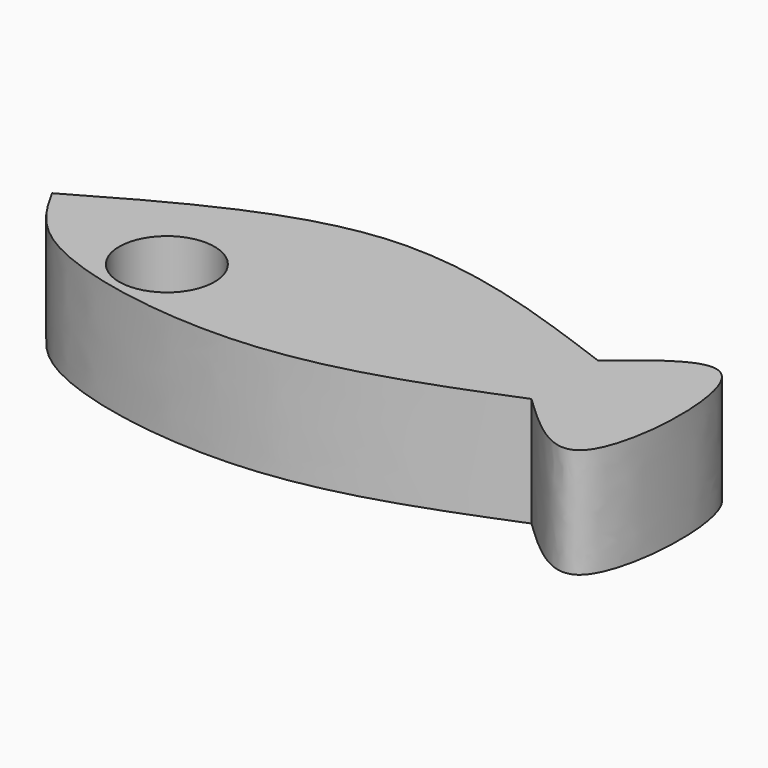
from build123d import *

# Parameters (mm, degrees)
F1_DEPTH = 11.684
F3_D     = 10.16


with BuildPart() as f1:
    # F0 (on Top) → F1 (new body)
    with BuildSketch(Plane.XY):
        with BuildLine():
            add(Edge.make_bspline(
                [(-36.1180268228, 4.0337503888), (-27.3021805537, 9.101057148), (-9.7698211862, 19.1785744295), (8.9001535273, 12.2858719608), (18.1822516024, 8.8590467349)],
                knots=[0, 0, 0, 0, 0.5028328523, 1, 1, 1, 1], degree=3))
            add(Edge.make_bspline(
                [(-36.1180268228, 4.0337503888), (-34.7839596362, 1.6128883032), (-31.2635443087, -4.7754256271), (-5.5172595701, -9.5463141676), (10.1612689912, -3.2309029238), (18.1822516024, 0)],
                knots=[0, 0, 0, 0, 0.2295947399, 0.6058681674, 1, 1, 1, 1], degree=3))
            add(Edge.make_bspline(
                [(18.1822516024, 8.8590467349), (22.0562457427, 12.1275590602), (30.9221363084, 19.6077646412), (29.7113094866, -10.9758153664), (21.6541939321, -3.3053349507), (18.1822516024, 0)],
                knots=[0, 0, 0, 0, 0.3063461125, 0.7010932414, 1, 1, 1, 1], degree=3))
        make_face()
    extrude(amount=F1_DEPTH)

    # F3 (through all)
    with Locations(Plane(origin=(0, 0, 0), x_dir=(1, 0, 0), z_dir=(0, 0, -1))):
        with Locations((-20.6633824855, 0)):
            Hole(F3_D / 2)


solid = f1.part
